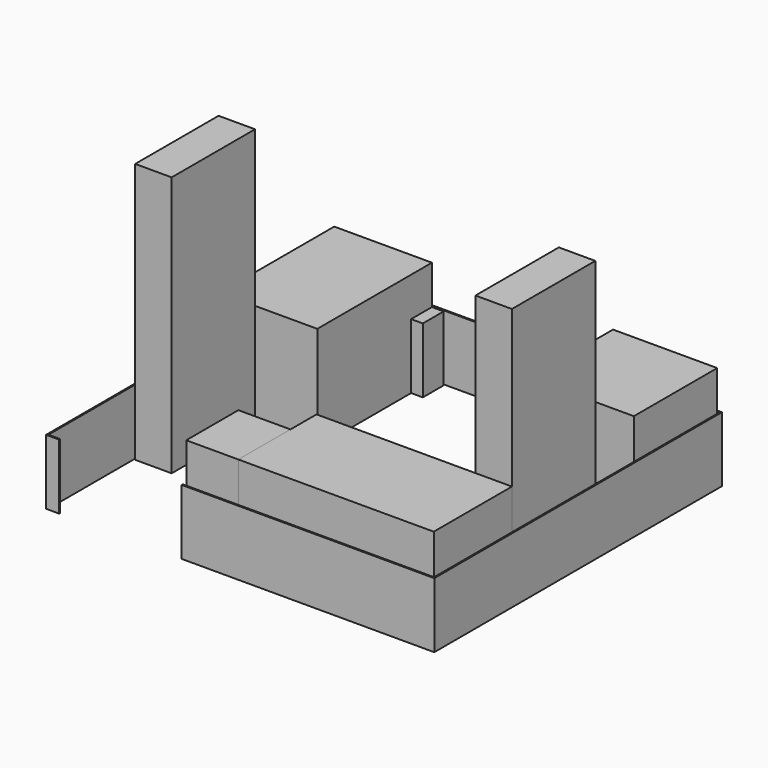
from build123d import *

# Parameters (mm, degrees)
F1_DEPTH = 500
F0_W     = 280
F0_H     = 800
F2_DEPTH = 2000
F0_W_2   = 90
F0_H_2   = 200
F3_DEPTH = 500
F0_W_3   = 670
F4_DEPTH = 800
F5_DEPTH = 800
F6_DEPTH = 2000
F0_W_4   = 800
F7_DEPTH = 800
F0_W_5   = 400
F0_H_3   = 500
F8_DEPTH = 800


with BuildPart() as f1:
    # F0 (on Top) → F1 (new body)
    with BuildSketch(Plane.XY):
        Polygon((-1490, -750), (-1490, 1990), (1470, 1990), (1470, -750), (-460, -750), (-460, -760), (1480, -760), (1480, 2000), (-1500, 2000), (-1500, -760), (-1400, -760), (-1400, -750), align=None)
    extrude(amount=F1_DEPTH)


with BuildPart() as f2:
    # F0 (on Top) → F2 (new body)
    with BuildSketch(Plane.XY):
        with Locations((-1340, 470)):
            Rectangle(F0_W, F0_H)
    extrude(amount=F2_DEPTH)


with BuildPart() as f3:
    # F0 (on Top) → F3 (new body)
    with BuildSketch(Plane.XY):
        with Locations((-685, 1880)):
            Rectangle(F0_W_2, F0_H_2)
    extrude(amount=F3_DEPTH)


with BuildPart() as f4:
    # F0 (on Top) → F4 (new body)
    with BuildSketch(Plane.XY):
        with Locations((-1065, 1880)):
            Rectangle(F0_W_3, F0_H_2)
        Polygon((-1400, 1780), (-1400, 1980), (-1480, 1980), (-1480, 880), (-730, 880), (-730, 1780), align=None)
    extrude(amount=F4_DEPTH)


with BuildPart() as f5:
    # F0 (on Top) → F5 (new body)
    with BuildSketch(Plane.XY):
        Polygon((1460, 10), (1180, 10), (-40, 10), (-40, -240), (-40, -740), (1460, -740), align=None)
    extrude(amount=F5_DEPTH)


with BuildPart() as f6:
    # F0 (on Top) → F6 (new body)
    with BuildSketch(Plane.XY):
        with Locations((1320, 410)):
            Rectangle(F0_W, F0_H)
    extrude(amount=F6_DEPTH)


with BuildPart() as f7:
    # F0 (on Top) → F7 (new body)
    with BuildSketch(Plane.XY):
        with Locations((1060, 1580)):
            Rectangle(F0_W_4, F0_H)
    extrude(amount=F7_DEPTH)


with BuildPart() as f8:
    # F0 (on Top) → F8 (new body)
    with BuildSketch(Plane.XY):
        with Locations((-240, -490)):
            Rectangle(F0_W_5, F0_H_3)
    extrude(amount=F8_DEPTH)


solid = Compound([f1.part, f2.part, f3.part, f4.part, f5.part, f6.part, f7.part, f8.part])
